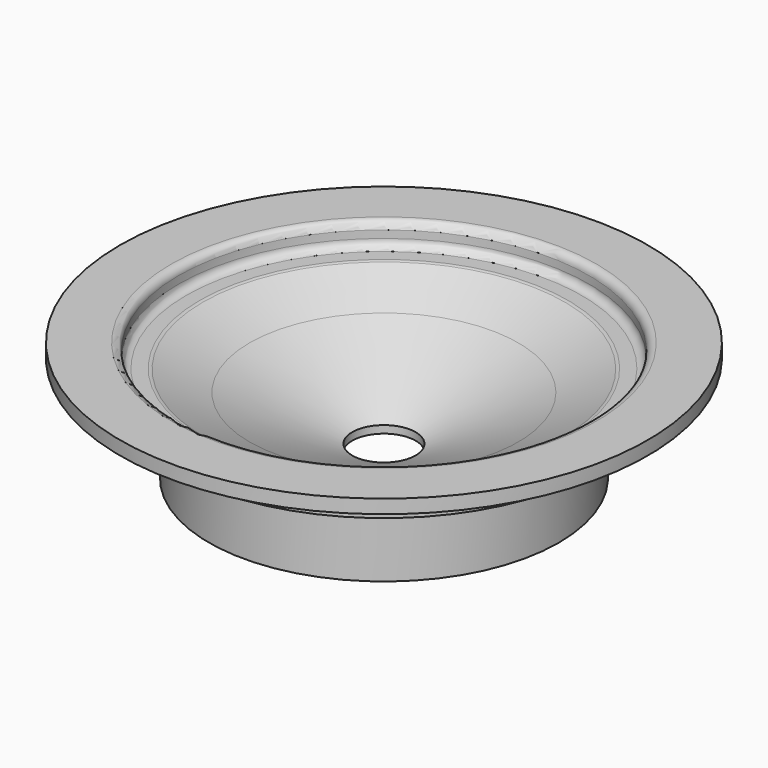
from build123d import *

# Parameters (mm, degrees)
F4_R = 0.5
F5_R = 0.5
F6_R = 0.5


# Not quite as in the source:
# - a feature of the source that left no trace in its solid (it failed there, or was rolled back) is left out


with BuildPart() as f1:
    # F0 (on Front) → F1 (revolve)
    with BuildSketch(Plane.XZ):
        Polygon((-2.1, -3), (-8.9066560708, 0), (-11.6, 0), (-11.6, -5), (-5.6, -5), (-5.6, -3.5), (-2.1, -3.5), align=None)
        Polygon((-11.6, 0), (-8.9066560708, 0), (-12.1, 1.4074505437), (-13.6, 1.4074505437), (-13.6, 2.9074505437), (-17.5, 2.9074505437), (-17.5, 2), (-14.1, 2), (-14.1, 0), align=None)
    revolve(axis=Axis((0, 0, -7.5), (0, 0, -1)))

    # F4
    f4_edges = [f1.edges().sort_by_distance(p)[0] for p in [
        (13.6, 0, 1.407451),
    ]]
    fillet(f4_edges, radius=F4_R)

    # F5
    f5_edges = [f1.edges().sort_by_distance(p)[0] for p in [
        (12.1, 0, 1.407451),
    ]]
    fillet(f5_edges, radius=F5_R)

    # F6
    f6_edges = [f1.edges().sort_by_distance(p)[0] for p in [
        (13.6, 0, 2.907451),
    ]]
    fillet(f6_edges, radius=F6_R)


solid = f1.part
